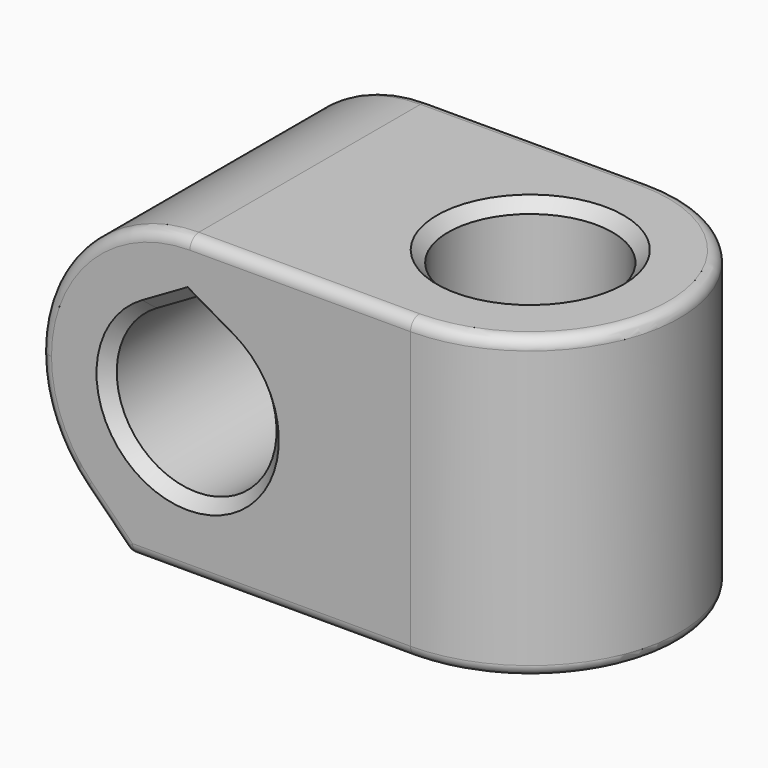
from build123d import *

# Parameters (mm, degrees)
F0_R     = 3.65
F1_DEPTH = 13.3
F3_DEPTH = 11
F4_R     = 6.65
F6_DEPTH = 25
F7_R     = 0.5
F8_SIZE  = 0.5


with BuildPart() as f1:
    # F0 (on Top) → F1 (new body)
    with BuildSketch(Plane.XY):
        with BuildLine():
            ThreePointArc((0, -6.65), (6.65, 0), (0, 6.65))
            Line((0, 6.65), (-16.45, 6.65))
            Line((-16.45, 6.65), (-16.45, -6.65))
            Line((-16.45, -6.65), (0, -6.65))
        make_face()
        with Locations((-9.8, 0)):
            Circle(F0_R, mode=Mode.SUBTRACT)
        Circle(F0_R, mode=Mode.SUBTRACT)
        with Locations((-9.8, 0)):
            Circle(F0_R)
    extrude(amount=F1_DEPTH)

    # F2 (on face) → F3 (cut)
    with BuildSketch(Plane.XZ.offset(6.65)):
        with BuildLine():
            Line((-9.9, 10.7491869112), (-11.675, 9.7243901834))
            ThreePointArc((-11.675, 9.7243901834), (-9.9, 3.1), (-8.125, 9.7243901834))
            Line((-8.125, 9.7243901834), (-9.9, 10.7491869112))
        make_face()
    extrude(amount=-F3_DEPTH, mode=Mode.SUBTRACT)

    # F4
    f4_edges = [f1.edges().sort_by_distance(p)[0] for p in [
        (-16.45, 0, 13.3),
    ]]
    fillet(f4_edges, radius=F4_R)

    # F5 (on face) → F6 (cut)
    with BuildSketch(Plane.XZ.offset(6.65)):
        with BuildLine():
            Line((-16.45, 0), (-12.5545201898, 0))
            Line((-12.5545201898, 0), (-14.5022600949, 1.9477399051))
            ThreePointArc((-14.5022600949, 1.9477399051), (-15.9437988912, 4.1051551748), (-16.45, 6.65))
            Line((-16.45, 6.65), (-16.45, 0))
        make_face()
    extrude(amount=-F6_DEPTH, mode=Mode.SUBTRACT)

    # F7
    f7_edges = [f1.edges().sort_by_distance(p)[0] for p in [
        (-4.9, -6.65, 13.3),
        (6.65, 0, 13.3),
        (-4.9, 6.65, 13.3),
        (-15.943799, 6.65, 9.194845),
        (-12.55452, 0, 0),
        (-13.52839, -6.65, 0.97387),
        (-6.27726, -6.65, 0),
        (6.65, 0, 0),
        (-15.943799, -6.65, 9.194845),
        (-6.27726, 6.65, 0),
        (-13.52839, 6.65, 0.97387),
    ]]
    fillet(f7_edges, radius=F7_R)

    # F8
    f8_edges = [f1.edges().sort_by_distance(p)[0] for p in [
        (-9.9, -6.65, 3.1),
        (-3.65, 0, 13.3),
        (-3.65, 0, 0),
        (-9.0125, -6.65, 10.236789),
        (-10.7875, -6.65, 10.236789),
    ]]
    chamfer(f8_edges, length=F8_SIZE)


solid = f1.part
